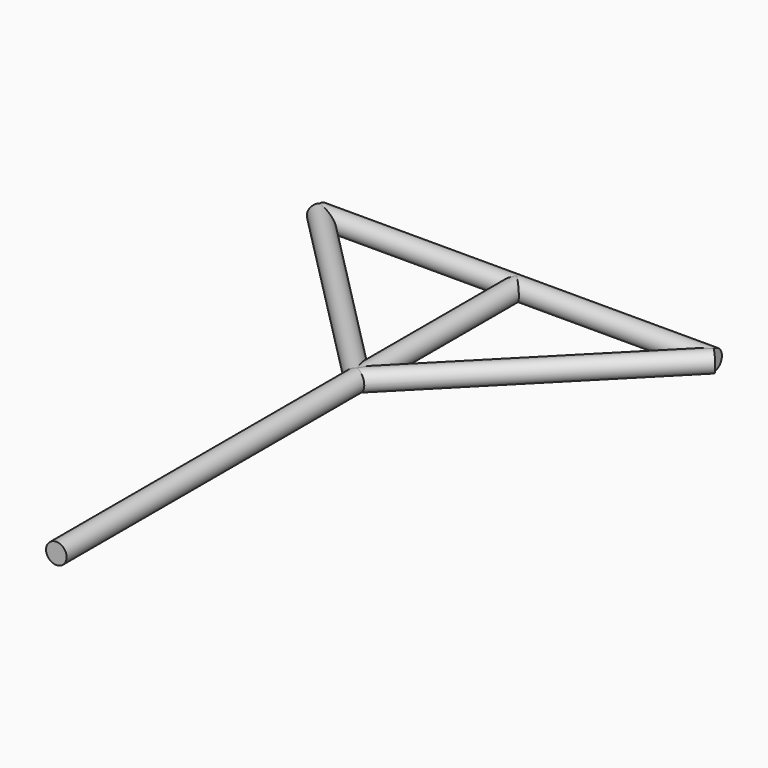
from build123d import *

# Parameters (mm, degrees)
F1_E1_W  = 76.2
F1_E1_H  = 3.9751
F3_E0_W  = 76.2
F3_E0_H  = 3.9751
F5_E3_W  = 108.4099765605
F5_E3_H  = 3.9751
F7_E2_W  = 108.4099765605
F7_E2_H  = 3.9751
F9_E4_W  = 77.1121457219
F9_E4_H  = 3.9751
F11_E5_W = 145.6045582891
F11_E5_H = 3.9751


with BuildPart() as f2:
    # F1_E1 (on explicit) → F2 (revolve)
    with BuildSketch(Plane(origin=(0, 0, 0), x_dir=(-1, 0, 0), z_dir=(0, 1, 0))):
        with Locations((38.1, 1.98755)):
            Rectangle(F1_E1_W, F1_E1_H)
    revolve(axis=Axis((-38.1, 0, 0), (-1, 0, 0)))

    # F3_E0 (on explicit) → F4 (revolve)
    with BuildSketch(Plane.XZ):
        with Locations((38.1, 1.98755)):
            Rectangle(F3_E0_W, F3_E0_H)
    revolve(axis=Axis((38.1, 0, 0), (1, 0, 0)))

    # F5_E3 (on explicit) → F6 (revolve)
    with BuildSketch(Plane(origin=(0, -77.1121457219, 0), x_dir=(0.7028873395, 0.7113011936, 0), z_dir=(0.7113011936, -0.7028873395, 0))):
        with Locations((54.2049882802, 1.98755)):
            Rectangle(F5_E3_W, F5_E3_H)
    revolve(axis=Axis((38.1, -38.556072861, 0), (0.7028873395, 0.7113011936, 0)))

    # F7_E2 (on explicit) → F8 (revolve)
    with BuildSketch(Plane(origin=(-76.2, 0, 0), x_dir=(0.7028873395, -0.7113011936, 0), z_dir=(-0.7113011936, -0.7028873395, 0))):
        with Locations((54.2049882802, 1.98755)):
            Rectangle(F7_E2_W, F7_E2_H)
    revolve(axis=Axis((-38.1, -38.556072861, 0), (0.7028873395, -0.7113011936, 0)))

    # F9_E4 (on explicit) → F10 (revolve)
    with BuildSketch(Plane(origin=(0, 0, 0), x_dir=(0, -1, 0), z_dir=(-1, 0, 0))):
        with Locations((38.556072861, 1.98755)):
            Rectangle(F9_E4_W, F9_E4_H)
    revolve(axis=Axis((0, -38.556072861, 0), (0, -1, 0)))

    # F11_E5 (on explicit) → F12 (revolve)
    with BuildSketch(Plane(origin=(0, -77.1121457219, 0), x_dir=(0, -1, 0), z_dir=(-1, 0, 0))):
        with Locations((72.8022791445, 1.98755)):
            Rectangle(F11_E5_W, F11_E5_H)
    revolve(axis=Axis((0, -149.9144248664, 0), (0, -1, 0)))


solid = f2.part
